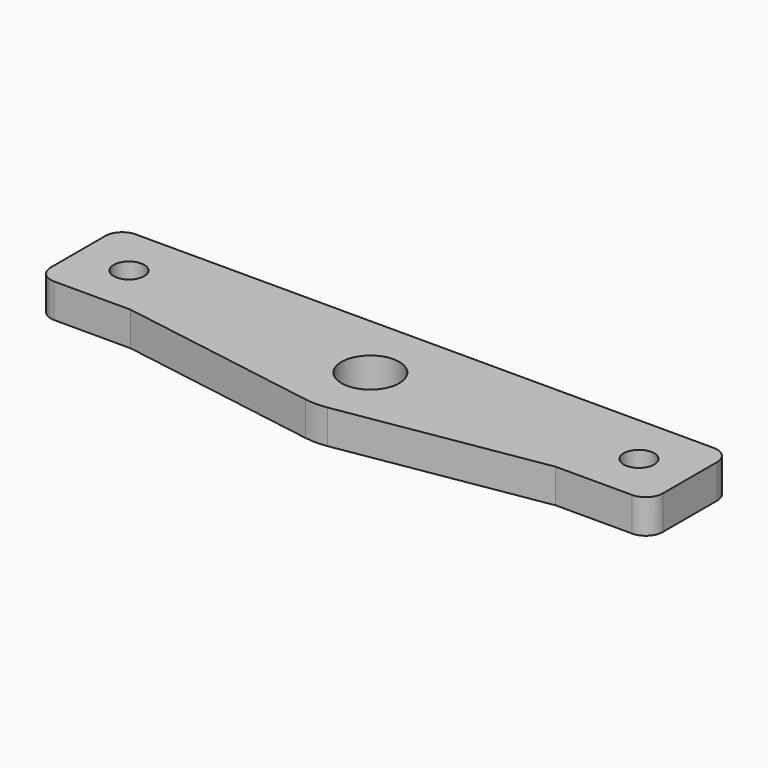
from build123d import *

# Parameters (mm, degrees)
F0_R     = 4.5
F0_R_2   = 8.5
F1_DEPTH = 10
F2_R     = 5


with BuildPart() as f1:
    # F0 (on Top) → F1 (new body)
    with BuildSketch(Plane.XY):
        with BuildLine():
            Line((-90, 20), (-90, -10))
            Line((-90, -10), (-62.5, -10))
            Line((-62.5, -10), (-17.3205080757, -10))
            ThreePointArc((-17.3205080757, -10), (-17.3205080604, 10.0000000264), (6.11e-08, 20))
            Line((6.11e-08, 20), (-90, 20))
        make_face()
        with Locations((-75, 5)):
            Circle(F0_R, mode=Mode.SUBTRACT)
        with BuildLine():
            Line((-17.3205080757, -10), (-62.5, -10))
            Line((-62.5, -10), (-3.2423308207, -19.7354323705))
            ThreePointArc((-3.2423308207, -19.7354323705), (-11.3755108338, -16.4498557219), (-17.3205080757, -10))
        make_face()
        with BuildLine():
            ThreePointArc((6.11e-08, 20), (-17.3205080604, 10.0000000264), (-17.3205080757, -10))
            Line((-17.3205080757, -10), (17.3205080757, -10))
            ThreePointArc((17.3205080757, -10), (19.3185165258, -5.1763809021), (20, 0))
            ThreePointArc((20, 0), (14.1421356453, 14.1421356021), (6.11e-08, 20))
        make_face()
        Circle(F0_R_2, mode=Mode.SUBTRACT)
        with BuildLine():
            Line((17.3205080757, -10), (-17.3205080757, -10))
            ThreePointArc((-17.3205080757, -10), (-11.3755108338, -16.4498557219), (-3.2423308207, -19.7354323705))
            ThreePointArc((-3.2423308207, -19.7354323705), (0, -20), (3.2423308207, -19.7354323705))
            ThreePointArc((3.2423308207, -19.7354323705), (11.3755108338, -16.4498557219), (17.3205080757, -10))
        make_face()
        with BuildLine():
            Line((90, 20), (6.11e-08, 20))
            ThreePointArc((6.11e-08, 20), (14.1421356453, 14.1421356021), (20, 0))
            ThreePointArc((20, 0), (19.3185165258, -5.1763809021), (17.3205080757, -10))
            Line((17.3205080757, -10), (62.5, -10))
            Line((62.5, -10), (90, -10))
            Line((90, -10), (90, 20))
        make_face()
        with Locations((75, 5)):
            Circle(F0_R, mode=Mode.SUBTRACT)
        with BuildLine():
            Line((62.5, -10), (17.3205080757, -10))
            ThreePointArc((17.3205080757, -10), (11.3755108338, -16.4498557219), (3.2423308207, -19.7354323705))
            Line((3.2423308207, -19.7354323705), (62.5, -10))
        make_face()
    extrude(amount=F1_DEPTH)

    # F2
    f2_edges = [f1.edges().sort_by_distance(p)[0] for p in [
        (-90, -10, 5),
        (90, -10, 5),
        (-90, 20, 5),
        (90, 20, 5),
    ]]
    fillet(f2_edges, radius=F2_R)


solid = f1.part
